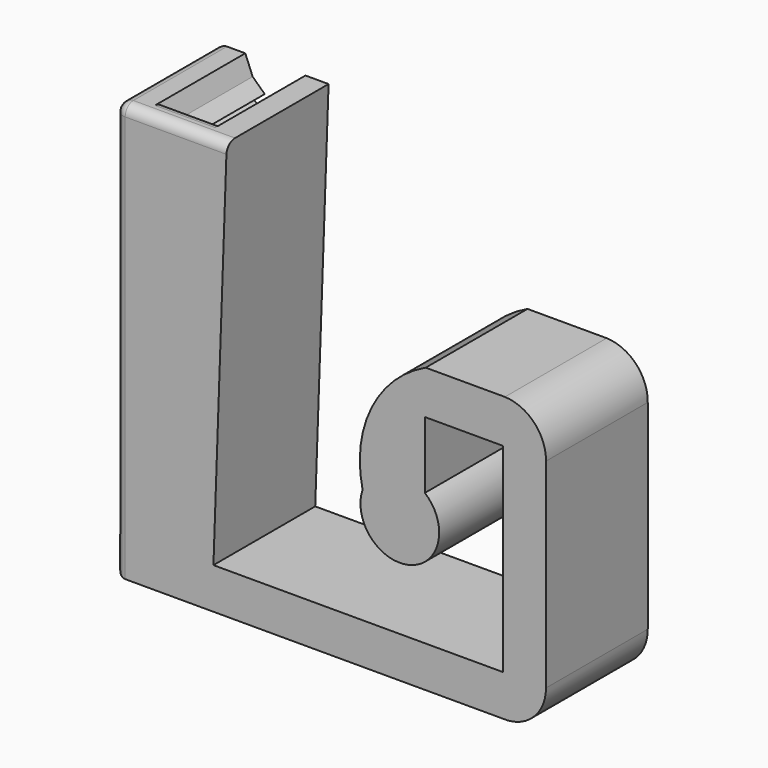
from build123d import *

# Parameters (mm, degrees)
F1_DEPTH = 5
F3_DEPTH = 1.2
F4_R     = 0.5
F5_R     = 0.5


# Not quite as in the source:
# - a feature names something its author has since deleted; it is built from what else it names


with BuildPart() as f1:
    # F0 (on Front) → F1 (new body)
    with BuildSketch(Plane.XZ):
        with BuildLine():
            Line((-14.8212344469, -7.0536743234), (-28.9212344469, -7.0536743234))
            Line((-28.9212344469, -7.0536743234), (-28.2704247986, 11.2749813125))
            Line((-28.2704247986, 11.2749813125), (-28.9218110621, 11.2749813125))
            Line((-28.9218110621, 11.2749813125), (-29.3961446732, 11.2749813125))
            Line((-29.3961446732, 11.2749813125), (-30.0026237965, 10.4798590764))
            Line((-30.0026237965, 10.4798590764), (-30.4116010666, 10.0127095357))
            Line((-30.4116010666, 10.0127095357), (-29.8413168639, 9.5870485529))
            Line((-29.8413168639, 9.5870485529), (-30.4648373276, 8.9966477826))
            Line((-30.4648373276, 8.9966477826), (-30.1126744598, 8.5086580366))
            Line((-30.1126744598, 8.5086580366), (-30.7294670492, 7.841065526))
            Line((-30.7294670492, 7.841065526), (-29.9794543535, 7.3754815385))
            Line((-29.9794543535, 7.3754815385), (-30.6979243471, 6.6930544935))
            Line((-30.6979243471, 6.6930544935), (-30.0398971885, 6.3235382549))
            Line((-30.0398971885, 6.3235382549), (-30.7178553194, 5.4153422825))
            Line((-30.7178553194, 5.4153422825), (-30.1331207156, 4.8448727466))
            Line((-30.1331207156, 4.8448727466), (-30.6775290519, 3.9221365005))
            Line((-30.6775290519, 3.9221365005), (-30.0103500485, 3.5474810284))
            Line((-30.0103500485, 3.5474810284), (-30.8397468179, 2.6670382358))
            Line((-30.8397468179, 2.6670382358), (-30.092863366, 1.9921413623))
            Line((-30.092863366, 1.9921413623), (-30.8324787766, 1.3930242276))
            Line((-30.8324787766, 1.3930242276), (-30.1521252841, 0.8188846987))
            Line((-30.1521252841, 0.8188846987), (-30.7863112539, 0.2193431865))
            Line((-30.7863112539, 0.2193431865), (-30.2403476089, -0.3106002114))
            Line((-30.2403476089, -0.3106002114), (-30.7600591332, -0.7401480107))
            Line((-30.7600591332, -0.7401480107), (-30.2189867944, -1.1601685546))
            Line((-30.2189867944, -1.1601685546), (-30.697863549, -1.5337655786))
            Line((-30.697863549, -1.5337655786), (-30.272686854, -1.8727472052))
            Line((-30.272686854, -1.8727472052), (-30.6971091777, -2.2358004935))
            Line((-30.6971091777, -2.2358004935), (-30.2377268672, -2.5755497627))
            Line((-30.2377268672, -2.5755497627), (-30.6886751205, -2.9733050615))
            Line((-30.6886751205, -2.9733050615), (-30.3040016443, -3.1427361537))
            Line((-30.3040016443, -3.1427361537), (-30.6638516486, -3.4895907156))
            Line((-30.6638516486, -3.4895907156), (-30.5218110621, -3.6142014433))
            ThreePointArc((-30.5218110621, -3.6142014433), (-30.1374019423, -4.9418633416), (-30.1468068426, -6.3240239819))
            ThreePointArc((-30.1468068426, -6.3240239819), (-31.3218110621, -6.9525761479), (-32.4968152816, -6.3240239819))
            ThreePointArc((-32.4968152816, -6.3240239819), (-32.5062201819, -4.9418633416), (-32.1218110621, -3.6142014433))
            Line((-32.1218110621, -3.6142014433), (-32.4906222522, -3.3608889207))
            Line((-32.4906222522, -3.3608889207), (-31.8935625255, -3.1926007941))
            Line((-31.8935625255, -3.1926007941), (-32.4732549489, -2.725369297))
            Line((-32.4732549489, -2.725369297), (-31.8681225181, -2.469912637))
            Line((-31.8681225181, -2.469912637), (-32.3700606823, -2.1127404179))
            Line((-32.3700606823, -2.1127404179), (-31.7923054099, -1.7308852402))
            Line((-31.7923054099, -1.7308852402), (-32.3993675411, -1.1372548761))
            Line((-32.3993675411, -1.1372548761), (-31.787391752, -0.9133979911))
            Line((-31.787391752, -0.9133979911), (-32.2625972331, -0.3995953302))
            Line((-32.2625972331, -0.3995953302), (-31.7277535796, -0.0062950298))
            Line((-31.7277535796, -0.0062950298), (-32.307446003, 0.4609364551))
            Line((-32.307446003, 0.4609364551), (-31.6469706595, 0.8653931436))
            Line((-31.6469706595, 0.8653931436), (-32.2801508009, 1.3617775403))
            Line((-32.2801508009, 1.3617775403), (-31.6663235426, 1.7637870042))
            Line((-31.6663235426, 1.7637870042), (-32.2516188025, 2.381386701))
            Line((-32.2516188025, 2.381386701), (-31.5948762, 2.771951491))
            Line((-31.5948762, 2.771951491), (-32.0806577802, 3.3034612425))
            Line((-32.0806577802, 3.3034612425), (-31.5831229091, 3.5578387324))
            Line((-31.5831229091, 3.5578387324), (-32.0962779224, 4.2157475837))
            Line((-32.0962779224, 4.2157475837), (-31.4544551075, 4.5507424511))
            Line((-31.4544551075, 4.5507424511), (-32.0472158492, 5.1405578852))
            Line((-32.0472158492, 5.1405578852), (-31.4172059298, 5.3744916804))
            Line((-31.4172059298, 5.3744916804), (-31.9610573351, 5.7992665097))
            Line((-31.9610573351, 5.7992665097), (-31.5387845039, 6.1167036183))
            Line((-31.5387845039, 6.1167036183), (-31.9445021451, 6.4705028199))
            Line((-31.9445021451, 6.4705028199), (-31.3227176666, 6.8809650838))
            Line((-31.3227176666, 6.8809650838), (-32.0109948516, 7.44209392))
            Line((-32.0109948516, 7.44209392), (-31.3543491066, 7.9823648557))
            Line((-31.3543491066, 7.9823648557), (-31.9620929658, 8.4623992443))
            Line((-31.9620929658, 8.4623992443), (-31.3818305731, 9.0230396017))
            Line((-31.3818305731, 9.0230396017), (-31.9348983467, 9.4317272305))
            Line((-31.9348983467, 9.4317272305), (-31.3805788755, 9.8327174783))
            Line((-31.3805788755, 9.8327174783), (-31.9697335362, 10.3881815448))
            Line((-31.9697335362, 10.3881815448), (-32.3277190328, 11.2749813125))
            Line((-32.3277190328, 11.2749813125), (-33.7218110621, 11.2749813125))
            Line((-33.7218110621, 11.2749813125), (-33.7218110621, -9.0536743234))
            Line((-33.7218110621, -9.0536743234), (-14.8212344469, -9.0536743234))
            ThreePointArc((-14.8212344469, -9.0536743234), (-13.3381540877, -8.5073007085), (-12.7176528294, -7.0536743234))
            Line((-12.7176528294, -7.0536743234), (-12.7176528294, 2.67616936))
            ThreePointArc((-12.7176528294, 2.67616936), (-13.2872120436, 4.138004008), (-14.7182294446, 4.7810805465))
            Line((-14.7182294446, 4.7810805465), (-18.5773239742, 4.7810805465))
            ThreePointArc((-18.5773239742, 4.7810805465), (-21.2175552856, 2.2046060367), (-21.6524992138, -1.4587074984))
            ThreePointArc((-21.6524992138, -1.4587074984), (-19.3188346891, -3.9296286003), (-18.6177780154, -0.6039766724))
            Line((-18.6177780154, -0.6039766724), (-18.6177780154, 2.6510965993))
            Line((-18.6177780154, 2.6510965993), (-14.8212344469, 2.6510965993))
            Line((-14.8212344469, 2.6510965993), (-14.8212344469, -7.0536743234))
        make_face()
    extrude(amount=F1_DEPTH)

    # F2 (on face) → F3 (join)
    with BuildSketch(Plane.XZ.offset(5)):
        with BuildLine():
            Line((-32.6968152816, 11.2749813125), (-32.6968152816, -7.0536743234))
            Line((-32.6968152816, -7.0536743234), (-29.3961446732, -7.0536743234))
            Line((-29.3961446732, -7.0536743234), (-29.3961446732, 11.2749813125))
            Line((-29.3961446732, 11.2749813125), (-30.0026237965, 10.4798590764))
            Line((-30.0026237965, 10.4798590764), (-30.4116010666, 10.0127095357))
            Line((-30.4116010666, 10.0127095357), (-29.8413168639, 9.5870485529))
            Line((-29.8413168639, 9.5870485529), (-30.4648373276, 8.9966477826))
            Line((-30.4648373276, 8.9966477826), (-30.1126744598, 8.5086580366))
            Line((-30.1126744598, 8.5086580366), (-30.7294670492, 7.841065526))
            Line((-30.7294670492, 7.841065526), (-29.9794543535, 7.3754815385))
            Line((-29.9794543535, 7.3754815385), (-30.6979243471, 6.6930544935))
            Line((-30.6979243471, 6.6930544935), (-30.0398971885, 6.3235382549))
            Line((-30.0398971885, 6.3235382549), (-30.7178553194, 5.4153422825))
            Line((-30.7178553194, 5.4153422825), (-30.1331207156, 4.8448727466))
            Line((-30.1331207156, 4.8448727466), (-30.6775290519, 3.9221365005))
            Line((-30.6775290519, 3.9221365005), (-30.0103500485, 3.5474810284))
            Line((-30.0103500485, 3.5474810284), (-30.8397468179, 2.6670382358))
            Line((-30.8397468179, 2.6670382358), (-30.092863366, 1.9921413623))
            Line((-30.092863366, 1.9921413623), (-30.8324787766, 1.3930242276))
            Line((-30.8324787766, 1.3930242276), (-30.1521252841, 0.8188846987))
            Line((-30.1521252841, 0.8188846987), (-30.7863112539, 0.2193431865))
            Line((-30.7863112539, 0.2193431865), (-30.2403476089, -0.3106002114))
            Line((-30.2403476089, -0.3106002114), (-30.7600591332, -0.7401480107))
            Line((-30.7600591332, -0.7401480107), (-30.2189867944, -1.1601685546))
            Line((-30.2189867944, -1.1601685546), (-30.697863549, -1.5337655786))
            Line((-30.697863549, -1.5337655786), (-30.272686854, -1.8727472052))
            Line((-30.272686854, -1.8727472052), (-30.6971091777, -2.2358004935))
            Line((-30.6971091777, -2.2358004935), (-30.2377268672, -2.5755497627))
            Line((-30.2377268672, -2.5755497627), (-30.6886751205, -2.9733050615))
            Line((-30.6886751205, -2.9733050615), (-30.3040016443, -3.1427361537))
            Line((-30.3040016443, -3.1427361537), (-30.6638516486, -3.4895907156))
            Line((-30.6638516486, -3.4895907156), (-30.5218110621, -3.6142014433))
            ThreePointArc((-30.5218110621, -3.6142014433), (-30.1374019423, -4.9418633416), (-30.1468068426, -6.3240239819))
            ThreePointArc((-30.1468068426, -6.3240239819), (-31.3218110621, -6.9525761479), (-32.4968152816, -6.3240239819))
            ThreePointArc((-32.4968152816, -6.3240239819), (-32.5062201819, -4.9418633416), (-32.1218110621, -3.6142014433))
            Line((-32.1218110621, -3.6142014433), (-32.4906222522, -3.3608889207))
            Line((-32.4906222522, -3.3608889207), (-31.8935625255, -3.1926007941))
            Line((-31.8935625255, -3.1926007941), (-32.4732549489, -2.725369297))
            Line((-32.4732549489, -2.725369297), (-31.8681225181, -2.469912637))
            Line((-31.8681225181, -2.469912637), (-32.3700606823, -2.1127404179))
            Line((-32.3700606823, -2.1127404179), (-31.7923054099, -1.7308852402))
            Line((-31.7923054099, -1.7308852402), (-32.3993675411, -1.1372548761))
            Line((-32.3993675411, -1.1372548761), (-31.787391752, -0.9133979911))
            Line((-31.787391752, -0.9133979911), (-32.2625972331, -0.3995953302))
            Line((-32.2625972331, -0.3995953302), (-31.7277535796, -0.0062950298))
            Line((-31.7277535796, -0.0062950298), (-32.307446003, 0.4609364551))
            Line((-32.307446003, 0.4609364551), (-31.6469706595, 0.8653931436))
            Line((-31.6469706595, 0.8653931436), (-32.2801508009, 1.3617775403))
            Line((-32.2801508009, 1.3617775403), (-31.6663235426, 1.7637870042))
            Line((-31.6663235426, 1.7637870042), (-32.2516188025, 2.381386701))
            Line((-32.2516188025, 2.381386701), (-31.5948762, 2.771951491))
            Line((-31.5948762, 2.771951491), (-32.0806577802, 3.3034612425))
            Line((-32.0806577802, 3.3034612425), (-31.5831229091, 3.5578387324))
            Line((-31.5831229091, 3.5578387324), (-32.0962779224, 4.2157475837))
            Line((-32.0962779224, 4.2157475837), (-31.4544551075, 4.5507424511))
            Line((-31.4544551075, 4.5507424511), (-32.0472158492, 5.1405578852))
            Line((-32.0472158492, 5.1405578852), (-31.4172059298, 5.3744916804))
            Line((-31.4172059298, 5.3744916804), (-31.9610573351, 5.7992665097))
            Line((-31.9610573351, 5.7992665097), (-31.5387845039, 6.1167036183))
            Line((-31.5387845039, 6.1167036183), (-31.9445021451, 6.4705028199))
            Line((-31.9445021451, 6.4705028199), (-31.3227176666, 6.8809650838))
            Line((-31.3227176666, 6.8809650838), (-32.0109948516, 7.44209392))
            Line((-32.0109948516, 7.44209392), (-31.3543491066, 7.9823648557))
            Line((-31.3543491066, 7.9823648557), (-31.9620929658, 8.4623992443))
            Line((-31.9620929658, 8.4623992443), (-31.3818305731, 9.0230396017))
            Line((-31.3818305731, 9.0230396017), (-31.9348983467, 9.4317272305))
            Line((-31.9348983467, 9.4317272305), (-31.3805788755, 9.8327174783))
            Line((-31.3805788755, 9.8327174783), (-31.9697335362, 10.3881815448))
            Line((-31.9697335362, 10.3881815448), (-32.3277190328, 11.2749813125))
            Line((-32.3277190328, 11.2749813125), (-32.6968152816, 11.2749813125))
        make_face()
        with BuildLine():
            Line((-30.0026237965, 10.4798590764), (-29.3961446732, 11.2749813125))
            Line((-29.3961446732, 11.2749813125), (-32.3277190328, 11.2749813125))
            Line((-32.3277190328, 11.2749813125), (-31.9697335362, 10.3881815448))
            Line((-31.9697335362, 10.3881815448), (-31.3805788755, 9.8327174783))
            Line((-31.3805788755, 9.8327174783), (-31.9348983467, 9.4317272305))
            Line((-31.9348983467, 9.4317272305), (-31.3818305731, 9.0230396017))
            Line((-31.3818305731, 9.0230396017), (-31.9620929658, 8.4623992443))
            Line((-31.9620929658, 8.4623992443), (-31.3543491066, 7.9823648557))
            Line((-31.3543491066, 7.9823648557), (-32.0109948516, 7.44209392))
            Line((-32.0109948516, 7.44209392), (-31.3227176666, 6.8809650838))
            Line((-31.3227176666, 6.8809650838), (-31.9445021451, 6.4705028199))
            Line((-31.9445021451, 6.4705028199), (-31.5387845039, 6.1167036183))
            Line((-31.5387845039, 6.1167036183), (-31.9610573351, 5.7992665097))
            Line((-31.9610573351, 5.7992665097), (-31.4172059298, 5.3744916804))
            Line((-31.4172059298, 5.3744916804), (-32.0472158492, 5.1405578852))
            Line((-32.0472158492, 5.1405578852), (-31.4544551075, 4.5507424511))
            Line((-31.4544551075, 4.5507424511), (-32.0962779224, 4.2157475837))
            Line((-32.0962779224, 4.2157475837), (-31.5831229091, 3.5578387324))
            Line((-31.5831229091, 3.5578387324), (-32.0806577802, 3.3034612425))
            Line((-32.0806577802, 3.3034612425), (-31.5948762, 2.771951491))
            Line((-31.5948762, 2.771951491), (-32.2516188025, 2.381386701))
            Line((-32.2516188025, 2.381386701), (-31.6663235426, 1.7637870042))
            Line((-31.6663235426, 1.7637870042), (-32.2801508009, 1.3617775403))
            Line((-32.2801508009, 1.3617775403), (-31.6469706595, 0.8653931436))
            Line((-31.6469706595, 0.8653931436), (-32.307446003, 0.4609364551))
            Line((-32.307446003, 0.4609364551), (-31.7277535796, -0.0062950298))
            Line((-31.7277535796, -0.0062950298), (-32.2625972331, -0.3995953302))
            Line((-32.2625972331, -0.3995953302), (-31.787391752, -0.9133979911))
            Line((-31.787391752, -0.9133979911), (-32.3993675411, -1.1372548761))
            Line((-32.3993675411, -1.1372548761), (-31.7923054099, -1.7308852402))
            Line((-31.7923054099, -1.7308852402), (-32.3700606823, -2.1127404179))
            Line((-32.3700606823, -2.1127404179), (-31.8681225181, -2.469912637))
            Line((-31.8681225181, -2.469912637), (-32.4732549489, -2.725369297))
            Line((-32.4732549489, -2.725369297), (-31.8935625255, -3.1926007941))
            Line((-31.8935625255, -3.1926007941), (-32.4906222522, -3.3608889207))
            Line((-32.4906222522, -3.3608889207), (-32.1218110621, -3.6142014433))
            ThreePointArc((-32.1218110621, -3.6142014433), (-32.5062201819, -4.9418633416), (-32.4968152816, -6.3240239819))
            ThreePointArc((-32.4968152816, -6.3240239819), (-31.3218110621, -6.9525761479), (-30.1468068426, -6.3240239819))
            ThreePointArc((-30.1468068426, -6.3240239819), (-30.1374019423, -4.9418633416), (-30.5218110621, -3.6142014433))
            Line((-30.5218110621, -3.6142014433), (-30.6638516486, -3.4895907156))
            Line((-30.6638516486, -3.4895907156), (-30.3040016443, -3.1427361537))
            Line((-30.3040016443, -3.1427361537), (-30.6886751205, -2.9733050615))
            Line((-30.6886751205, -2.9733050615), (-30.2377268672, -2.5755497627))
            Line((-30.2377268672, -2.5755497627), (-30.6971091777, -2.2358004935))
            Line((-30.6971091777, -2.2358004935), (-30.272686854, -1.8727472052))
            Line((-30.272686854, -1.8727472052), (-30.697863549, -1.5337655786))
            Line((-30.697863549, -1.5337655786), (-30.2189867944, -1.1601685546))
            Line((-30.2189867944, -1.1601685546), (-30.7600591332, -0.7401480107))
            Line((-30.7600591332, -0.7401480107), (-30.2403476089, -0.3106002114))
            Line((-30.2403476089, -0.3106002114), (-30.7863112539, 0.2193431865))
            Line((-30.7863112539, 0.2193431865), (-30.1521252841, 0.8188846987))
            Line((-30.1521252841, 0.8188846987), (-30.8324787766, 1.3930242276))
            Line((-30.8324787766, 1.3930242276), (-30.092863366, 1.9921413623))
            Line((-30.092863366, 1.9921413623), (-30.8397468179, 2.6670382358))
            Line((-30.8397468179, 2.6670382358), (-30.0103500485, 3.5474810284))
            Line((-30.0103500485, 3.5474810284), (-30.6775290519, 3.9221365005))
            Line((-30.6775290519, 3.9221365005), (-30.1331207156, 4.8448727466))
            Line((-30.1331207156, 4.8448727466), (-30.7178553194, 5.4153422825))
            Line((-30.7178553194, 5.4153422825), (-30.0398971885, 6.3235382549))
            Line((-30.0398971885, 6.3235382549), (-30.6979243471, 6.6930544935))
            Line((-30.6979243471, 6.6930544935), (-29.9794543535, 7.3754815385))
            Line((-29.9794543535, 7.3754815385), (-30.7294670492, 7.841065526))
            Line((-30.7294670492, 7.841065526), (-30.1126744598, 8.5086580366))
            Line((-30.1126744598, 8.5086580366), (-30.4648373276, 8.9966477826))
            Line((-30.4648373276, 8.9966477826), (-29.8413168639, 9.5870485529))
            Line((-29.8413168639, 9.5870485529), (-30.4116010666, 10.0127095357))
            Line((-30.4116010666, 10.0127095357), (-30.0026237965, 10.4798590764))
        make_face()
        with BuildLine():
            Line((-29.3961446732, -7.0536743234), (-32.6968152816, -7.0536743234))
            Line((-32.6968152816, -7.0536743234), (-32.6968152816, 11.2749813125))
            Line((-32.6968152816, 11.2749813125), (-33.7218110621, 11.2749813125))
            Line((-33.7218110621, 11.2749813125), (-33.7218110621, -9.0536743234))
            Line((-33.7218110621, -9.0536743234), (-14.8212344469, -9.0536743234))
            ThreePointArc((-14.8212344469, -9.0536743234), (-13.3381540877, -8.5073007085), (-12.7176528294, -7.0536743234))
            Line((-12.7176528294, -7.0536743234), (-12.7176528294, 2.67616936))
            ThreePointArc((-12.7176528294, 2.67616936), (-13.2872120436, 4.138004008), (-14.7182294446, 4.7810805465))
            Line((-14.7182294446, 4.7810805465), (-18.5773239742, 4.7810805465))
            ThreePointArc((-18.5773239742, 4.7810805465), (-21.2175552856, 2.2046060367), (-21.6524992138, -1.4587074984))
            ThreePointArc((-21.6524992138, -1.4587074984), (-19.3188346891, -3.9296286003), (-18.6177780154, -0.6039766724))
            Line((-18.6177780154, -0.6039766724), (-18.6177780154, 2.6510965993))
            Line((-18.6177780154, 2.6510965993), (-14.8212344469, 2.6510965993))
            Line((-14.8212344469, 2.6510965993), (-14.8212344469, -7.0536743234))
            Line((-14.8212344469, -7.0536743234), (-28.9212344469, -7.0536743234))
            Line((-28.9212344469, -7.0536743234), (-28.2704247986, 11.2749813125))
            Line((-28.2704247986, 11.2749813125), (-29.3961446732, 11.2749813125))
            Line((-29.3961446732, 11.2749813125), (-29.3961446732, -7.0536743234))
        make_face()
    extrude(amount=F3_DEPTH)

    # F4
    f4_edges = [f1.edges().sort_by_distance(p)[0] for p in [
        (-30.861932, -5, 11.274981),
    ]]
    fillet(f4_edges, radius=F4_R)

    # F5
    f5_edges = [f1.edges().sort_by_distance(p)[0] for p in [
        (-33.721811, 0, 1.110653),
        (-33.721811, -6.2, 1.110653),
        (-33.721811, -3.1, -9.053674),
        (-30.996118, -6.2, 11.274981),
        (-33.721811, -3.1, 11.274981),
    ]]
    fillet(f5_edges, radius=F5_R)


solid = f1.part
